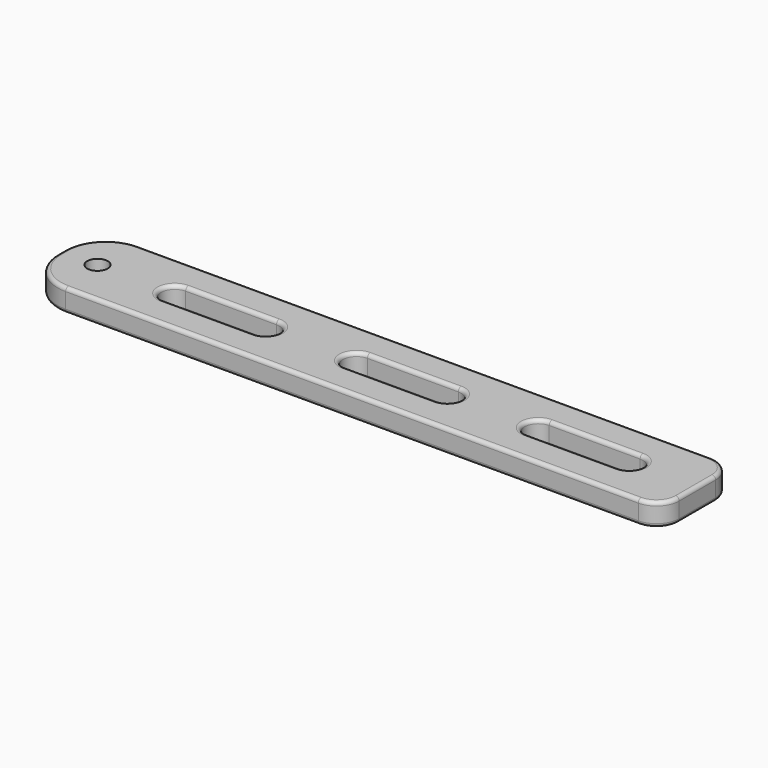
from build123d import *

# Parameters (mm, degrees)
F1_DEPTH = 5
F2_R     = 9
F3_R     = 5
F4_R     = 0.8
F5_R     = 2.25
F6_DEPTH = 25


# Not quite as in the source:
# - a feature names something its author has since deleted; it is built from what else it names


with BuildPart() as f1:
    # F0 (on Top) → F1 (new body)
    with BuildSketch(Plane.XY):
        with BuildLine():
            Line((64.1480287884, 35.2721845528), (-75.8519712116, 35.2721845528))
            Line((-75.8519712116, 35.2721845528), (-75.8519712116, 15.2721845528))
            Line((-75.8519712116, 15.2721845528), (64.1480287884, 15.2721845528))
            Line((64.1480287884, 15.2721845528), (64.1480287884, 22.2721845528))
            Line((64.1480287884, 22.2721845528), (49.148028803, 22.2721845528))
            Line((49.148028803, 22.2721845528), (29.1480287884, 22.2721845528))
            Line((29.1480287884, 22.2721845528), (9.1480287884, 22.2721845528))
            Line((9.1480287884, 22.2721845528), (-10.8519712116, 22.2721845528))
            Line((-10.8519712116, 22.2721845528), (-30.8519712116, 22.2721845528))
            Line((-30.8519712116, 22.2721845528), (-50.8519712116, 22.2721845528))
            ThreePointArc((-50.8519712116, 22.2721845528), (-53.8519712116, 25.2721845528), (-50.8519712116, 28.2721845528))
            Line((-50.8519712116, 28.2721845528), (-30.8519712116, 28.2721845528))
            Line((-30.8519712116, 28.2721845528), (-10.8519712116, 28.2721845528))
            Line((-10.8519712116, 28.2721845528), (9.1480288048, 28.2721845528))
            Line((9.1480288048, 28.2721845528), (29.1480287884, 28.2721845528))
            Line((29.1480287884, 28.2721845528), (49.1480287884, 28.2721845528))
            Line((49.1480287884, 28.2721845528), (64.1480287884, 28.2721845528))
            Line((64.1480287884, 28.2721845528), (64.1480287884, 35.2721845528))
        make_face()
        with BuildLine():
            Line((64.1480287884, 22.2721845528), (64.1480287884, 28.2721845528))
            Line((64.1480287884, 28.2721845528), (49.1480287884, 28.2721845528))
            ThreePointArc((49.1480287884, 28.2721845528), (51.269349132, 27.3935048963), (52.1480287884, 25.2721845528))
            ThreePointArc((52.1480287884, 25.2721845528), (51.2693491371, 23.1508642144), (49.148028803, 22.2721845528))
            Line((49.148028803, 22.2721845528), (64.1480287884, 22.2721845528))
        make_face()
        with BuildLine():
            ThreePointArc((29.1480287884, 22.2721845528), (26.1480287884, 25.2721845528), (29.1480287884, 28.2721845528))
            Line((29.1480287884, 28.2721845528), (9.1480288048, 28.2721845528))
            ThreePointArc((9.1480288048, 28.2721845528), (11.2693491378, 27.3935048905), (12.1480287884, 25.2721845528))
            ThreePointArc((12.1480287884, 25.2721845528), (11.269349132, 23.1508642092), (9.1480287884, 22.2721845528))
            Line((9.1480287884, 22.2721845528), (29.1480287884, 22.2721845528))
        make_face()
        with BuildLine():
            ThreePointArc((-10.8519712116, 22.2721845528), (-13.8519712116, 25.2721845528), (-10.8519712116, 28.2721845528))
            Line((-10.8519712116, 28.2721845528), (-30.8519712116, 28.2721845528))
            ThreePointArc((-30.8519712116, 28.2721845528), (-28.730650868, 27.3935048963), (-27.8519712116, 25.2721845528))
            ThreePointArc((-27.8519712116, 25.2721845528), (-28.730650868, 23.1508642092), (-30.8519712116, 22.2721845528))
            Line((-30.8519712116, 22.2721845528), (-10.8519712116, 22.2721845528))
        make_face()
    extrude(amount=F1_DEPTH)

    # F2
    f2_edges = [f1.edges().sort_by_distance(p)[0] for p in [
        (-75.851971, 35.272185, 2.5),
        (-75.851971, 15.272185, 2.5),
    ]]
    fillet(f2_edges, radius=F2_R)

    # F3
    f3_edges = [f1.edges().sort_by_distance(p)[0] for p in [
        (64.148029, 15.272185, 2.5),
        (64.148029, 35.272185, 2.5),
    ]]
    fillet(f3_edges, radius=F3_R)

    # F4
    f4_edges = [f1.edges().sort_by_distance(p)[0] for p in [
        (-13.851971, 25.272185, 5),
        (26.148029, 25.272185, 5),
        (-53.851971, 25.272185, 5),
        (26.148029, 25.272185, 0),
        (-13.851971, 25.272185, 0),
        (-53.851971, 25.272185, 0),
        (-3.851971, 15.272185, 5),
        (-3.851971, 15.272185, 0),
    ]]
    fillet(f4_edges, radius=F4_R)

    # F5 (on face) → F6 (cut)
    with BuildSketch(Plane.XY.offset(5)):
        with Locations((-67.8519712116, 25.2721845528)):
            Circle(F5_R)
    extrude(amount=-F6_DEPTH, mode=Mode.SUBTRACT)


solid = f1.part
